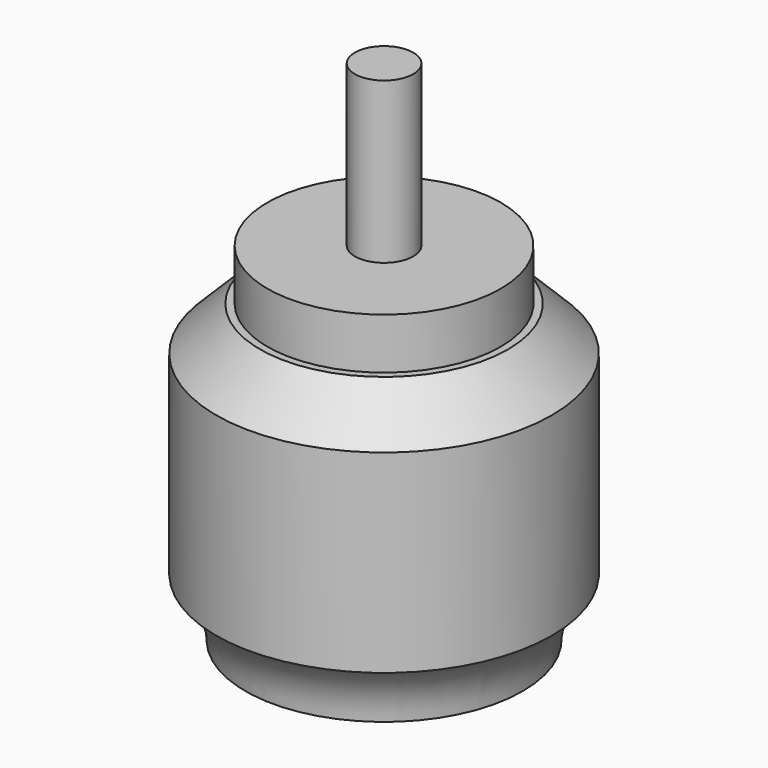
from build123d import *

# Parameters (mm, degrees)
F0_R     = 11.5
F1_DEPTH = 20.3
F2_R     = 11.5
F2_R_2   = 9.5
F3_DEPTH = 4
F5_DEPTH = 5
F6_SIZE  = 3
F7_R     = 2
F8_DEPTH = 14.5
F7_R_2   = 8
F9_DEPTH = 3.5


# Not quite as in the source:
# - a fillet or chamfer that OpenCascade refuses, or shapes differently, is made with other operations: its cross-section is extruded or revolved along the edge and cut away or added


with BuildPart() as f1:
    # F0 (on Top) → F1 (new body)
    with BuildSketch(Plane.XY):
        Circle(F0_R)
        with BuildLine():
            ThreePointArc((-7.9375, 0.9980449639), (0, 8), (7.9375, 0.9980449639))
            ThreePointArc((7.9375, 0.9980449639), (8.6846531969, 0.7288689869), (9, 0))
            ThreePointArc((9, 0), (8.6846531969, -0.7288689869), (7.9375, -0.9980449639))
            ThreePointArc((7.9375, -0.9980449639), (0, -8), (-7.9375, -0.9980449639))
            ThreePointArc((-7.9375, -0.9980449639), (-9, 0), (-7.9375, 0.9980449639))
        make_face(mode=Mode.SUBTRACT)
        with BuildLine():
            ThreePointArc((7.9375, 0.9980449639), (7.9843597113, 0.5), (8, 0))
            ThreePointArc((8, 0), (7.9843597113, -0.5), (7.9375, -0.9980449639))
            ThreePointArc((7.9375, -0.9980449639), (8.6846531969, -0.7288689869), (9, 0))
            ThreePointArc((9, 0), (8.6846531969, 0.7288689869), (7.9375, 0.9980449639))
        make_face()
        with BuildLine():
            ThreePointArc((7, 0), (7.2711310131, 0.6846531969), (7.9375, 0.9980449639))
            ThreePointArc((7.9375, 0.9980449639), (0, 8), (-7.9375, 0.9980449639))
            ThreePointArc((-7.9375, 0.9980449639), (-7.2711310131, 0.6846531969), (-7, 0))
            Line((-7, 0), (-6, 0))
            ThreePointArc((-6, 0), (-4.5814370219, 3.8743302407), (-0.9965217286, 5.9166666667))
            ThreePointArc((-0.9965217286, 5.9166666667), (-0.041702946, 6.9991300537), (1, 6))
            ThreePointArc((1, 6), (0.9991300537, 5.958297054), (0.9965217286, 5.9166666667))
            ThreePointArc((0.9965217286, 5.9166666667), (4.5814370219, 3.8743302407), (6, 0))
            Line((6, 0), (7, 0))
        make_face()
        with BuildLine():
            Line((0, 0), (6, 0))
            ThreePointArc((6, 0), (4.5814370219, 3.8743302407), (0.9965217286, 5.9166666667))
            ThreePointArc((0.9965217286, 5.9166666667), (0.6770032004, 5.2640199278), (0, 5))
            Line((0, 5), (0, 0))
        make_face()
        with BuildLine():
            Line((-6, 0), (0, 0))
            Line((0, 0), (0, 5))
            ThreePointArc((0, 5), (-0.6770032004, 5.2640199278), (-0.9965217286, 5.9166666667))
            ThreePointArc((-0.9965217286, 5.9166666667), (-4.5814370219, 3.8743302407), (-6, 0))
        make_face()
        with BuildLine():
            Line((0, -5), (0, 0))
            Line((0, 0), (-6, 0))
            ThreePointArc((-6, 0), (-4.5814370219, -3.8743302407), (-0.9965217286, -5.9166666667))
            ThreePointArc((-0.9965217286, -5.9166666667), (-0.6770032004, -5.2640199278), (0, -5))
        make_face()
        with BuildLine():
            ThreePointArc((0.9965217286, -5.9166666667), (4.5814370219, -3.8743302407), (6, 0))
            Line((6, 0), (0, 0))
            Line((0, 0), (0, -5))
            ThreePointArc((0, -5), (0.6770032004, -5.2640199278), (0.9965217286, -5.9166666667))
        make_face()
        with BuildLine():
            ThreePointArc((0, 5), (0.6770032004, 5.2640199278), (0.9965217286, 5.9166666667))
            ThreePointArc((0.9965217286, 5.9166666667), (0.5, 5.9791303716), (0, 6))
            Line((0, 6), (0, 5))
        make_face()
        with BuildLine():
            Line((0, 5), (0, 6))
            ThreePointArc((0, 6), (-0.5, 5.9791303716), (-0.9965217286, 5.9166666667))
            ThreePointArc((-0.9965217286, 5.9166666667), (-0.6770032004, 5.2640199278), (0, 5))
        make_face()
        with BuildLine():
            ThreePointArc((0, 6), (0.5, 5.9791303716), (0.9965217286, 5.9166666667))
            ThreePointArc((0.9965217286, 5.9166666667), (0.9991300537, 5.958297054), (1, 6))
            ThreePointArc((1, 6), (-0.041702946, 6.9991300537), (-0.9965217286, 5.9166666667))
            ThreePointArc((-0.9965217286, 5.9166666667), (-0.5, 5.9791303716), (0, 6))
        make_face()
        with BuildLine():
            ThreePointArc((7.9375, -0.9980449639), (7.9843597113, -0.5), (8, 0))
            Line((8, 0), (7, 0))
            ThreePointArc((7, 0), (7.2711310131, -0.6846531969), (7.9375, -0.9980449639))
        make_face()
        with BuildLine():
            Line((7, 0), (8, 0))
            ThreePointArc((8, 0), (7.9843597113, 0.5), (7.9375, 0.9980449639))
            ThreePointArc((7.9375, 0.9980449639), (7.2711310131, 0.6846531969), (7, 0))
        make_face()
        with BuildLine():
            ThreePointArc((-7.9375, -0.9980449639), (0, -8), (7.9375, -0.9980449639))
            ThreePointArc((7.9375, -0.9980449639), (7.2711310131, -0.6846531969), (7, 0))
            Line((7, 0), (6, 0))
            ThreePointArc((6, 0), (4.5814370219, -3.8743302407), (0.9965217286, -5.9166666667))
            ThreePointArc((0.9965217286, -5.9166666667), (0.9991300537, -5.958297054), (1, -6))
            ThreePointArc((1, -6), (-0.041702946, -6.9991300537), (-0.9965217286, -5.9166666667))
            ThreePointArc((-0.9965217286, -5.9166666667), (-4.5814370219, -3.8743302407), (-6, 0))
            Line((-6, 0), (-7, 0))
            ThreePointArc((-7, 0), (-7.2711310131, -0.6846531969), (-7.9375, -0.9980449639))
        make_face()
        with BuildLine():
            ThreePointArc((1, -6), (0.9991300537, -5.958297054), (0.9965217286, -5.9166666667))
            ThreePointArc((0.9965217286, -5.9166666667), (0.5, -5.9791303716), (0, -6))
            ThreePointArc((0, -6), (-0.5, -5.9791303716), (-0.9965217286, -5.9166666667))
            ThreePointArc((-0.9965217286, -5.9166666667), (-0.041702946, -6.9991300537), (1, -6))
        make_face()
        with BuildLine():
            ThreePointArc((0, -6), (0.5, -5.9791303716), (0.9965217286, -5.9166666667))
            ThreePointArc((0.9965217286, -5.9166666667), (0.6770032004, -5.2640199278), (0, -5))
            Line((0, -5), (0, -6))
        make_face()
        with BuildLine():
            ThreePointArc((-0.9965217286, -5.9166666667), (-0.5, -5.9791303716), (0, -6))
            Line((0, -6), (0, -5))
            ThreePointArc((0, -5), (-0.6770032004, -5.2640199278), (-0.9965217286, -5.9166666667))
        make_face()
        with BuildLine():
            ThreePointArc((-8, 0), (-7.9843597113, -0.5), (-7.9375, -0.9980449639))
            ThreePointArc((-7.9375, -0.9980449639), (-7.2711310131, -0.6846531969), (-7, 0))
            Line((-7, 0), (-8, 0))
        make_face()
        with BuildLine():
            ThreePointArc((-8, 0), (-7.9843597113, 0.5), (-7.9375, 0.9980449639))
            ThreePointArc((-7.9375, 0.9980449639), (-9, 0), (-7.9375, -0.9980449639))
            ThreePointArc((-7.9375, -0.9980449639), (-7.9843597113, -0.5), (-8, 0))
        make_face()
        with BuildLine():
            ThreePointArc((-7, 0), (-7.2711310131, 0.6846531969), (-7.9375, 0.9980449639))
            ThreePointArc((-7.9375, 0.9980449639), (-7.9843597113, 0.5), (-8, 0))
            Line((-8, 0), (-7, 0))
        make_face()
    extrude(amount=F1_DEPTH)

    # F2 (on face) → F3 (cut)
    with BuildSketch(Plane(origin=(0, 0, 0), x_dir=(1, 0, 0), z_dir=(0, 0, -1))):
        Circle(F2_R)
        Circle(F2_R_2, mode=Mode.SUBTRACT)
    extrude(amount=-F3_DEPTH, mode=Mode.SUBTRACT)

    # F4: fillet of radius 5 on 1 edges, made by hand

    # F4_s1 → F4_t2 (revolve)
    with BuildSketch(Plane.XZ):
        with BuildLine():
            ThreePointArc((11.5, 4), (10.027864045, 2.2360679775), (9.5, 0))
            Line((9.5, 0), (9.5, 4))
            Line((9.5, 4), (11.5, 4))
        make_face()
    revolve(axis=Axis((0, 0, 4), (0, 0, -1)))

    # F0 (on Top) → F5 (cut)
    with BuildSketch(Plane.XY):
        with BuildLine():
            ThreePointArc((-8, 0), (-7.9843597113, 0.5), (-7.9375, 0.9980449639))
            ThreePointArc((-7.9375, 0.9980449639), (-9, 0), (-7.9375, -0.9980449639))
            ThreePointArc((-7.9375, -0.9980449639), (-7.9843597113, -0.5), (-8, 0))
        make_face()
        with BuildLine():
            ThreePointArc((-8, 0), (-7.9843597113, -0.5), (-7.9375, -0.9980449639))
            ThreePointArc((-7.9375, -0.9980449639), (-7.2711310131, -0.6846531969), (-7, 0))
            Line((-7, 0), (-8, 0))
        make_face()
        with BuildLine():
            ThreePointArc((-7, 0), (-7.2711310131, 0.6846531969), (-7.9375, 0.9980449639))
            ThreePointArc((-7.9375, 0.9980449639), (-7.9843597113, 0.5), (-8, 0))
            Line((-8, 0), (-7, 0))
        make_face()
        with BuildLine():
            ThreePointArc((0, 6), (0.5, 5.9791303716), (0.9965217286, 5.9166666667))
            ThreePointArc((0.9965217286, 5.9166666667), (0.9991300537, 5.958297054), (1, 6))
            ThreePointArc((1, 6), (-0.041702946, 6.9991300537), (-0.9965217286, 5.9166666667))
            ThreePointArc((-0.9965217286, 5.9166666667), (-0.5, 5.9791303716), (0, 6))
        make_face()
        with BuildLine():
            ThreePointArc((0, 5), (0.6770032004, 5.2640199278), (0.9965217286, 5.9166666667))
            ThreePointArc((0.9965217286, 5.9166666667), (0.5, 5.9791303716), (0, 6))
            Line((0, 6), (0, 5))
        make_face()
        with BuildLine():
            Line((0, 5), (0, 6))
            ThreePointArc((0, 6), (-0.5, 5.9791303716), (-0.9965217286, 5.9166666667))
            ThreePointArc((-0.9965217286, 5.9166666667), (-0.6770032004, 5.2640199278), (0, 5))
        make_face()
        with BuildLine():
            ThreePointArc((7.9375, 0.9980449639), (7.9843597113, 0.5), (8, 0))
            ThreePointArc((8, 0), (7.9843597113, -0.5), (7.9375, -0.9980449639))
            ThreePointArc((7.9375, -0.9980449639), (8.6846531969, -0.7288689869), (9, 0))
            ThreePointArc((9, 0), (8.6846531969, 0.7288689869), (7.9375, 0.9980449639))
        make_face()
        with BuildLine():
            ThreePointArc((7.9375, -0.9980449639), (7.9843597113, -0.5), (8, 0))
            Line((8, 0), (7, 0))
            ThreePointArc((7, 0), (7.2711310131, -0.6846531969), (7.9375, -0.9980449639))
        make_face()
        with BuildLine():
            Line((7, 0), (8, 0))
            ThreePointArc((8, 0), (7.9843597113, 0.5), (7.9375, 0.9980449639))
            ThreePointArc((7.9375, 0.9980449639), (7.2711310131, 0.6846531969), (7, 0))
        make_face()
        with BuildLine():
            ThreePointArc((1, -6), (0.9991300537, -5.958297054), (0.9965217286, -5.9166666667))
            ThreePointArc((0.9965217286, -5.9166666667), (0.5, -5.9791303716), (0, -6))
            ThreePointArc((0, -6), (-0.5, -5.9791303716), (-0.9965217286, -5.9166666667))
            ThreePointArc((-0.9965217286, -5.9166666667), (-0.041702946, -6.9991300537), (1, -6))
        make_face()
        with BuildLine():
            ThreePointArc((-0.9965217286, -5.9166666667), (-0.5, -5.9791303716), (0, -6))
            Line((0, -6), (0, -5))
            ThreePointArc((0, -5), (-0.6770032004, -5.2640199278), (-0.9965217286, -5.9166666667))
        make_face()
        with BuildLine():
            ThreePointArc((0, -6), (0.5, -5.9791303716), (0.9965217286, -5.9166666667))
            ThreePointArc((0.9965217286, -5.9166666667), (0.6770032004, -5.2640199278), (0, -5))
            Line((0, -5), (0, -6))
        make_face()
    extrude(amount=F5_DEPTH, mode=Mode.SUBTRACT)

    # F6
    f6_edges = [f1.edges().sort_by_distance(p)[0] for p in [
        (-11.5, 0, 20.3),
    ]]
    chamfer(f6_edges, length=F6_SIZE)

    # F7 (on face) → F8 (join)
    with BuildSketch(Plane.XY.offset(20.3)):
        Circle(F7_R)
    extrude(amount=F8_DEPTH)

    # F7 (on face) → F9 (join)
    with BuildSketch(Plane.XY.offset(20.3)):
        Circle(F7_R_2)
        Circle(F7_R, mode=Mode.SUBTRACT)
    extrude(amount=F9_DEPTH)


solid = f1.part
